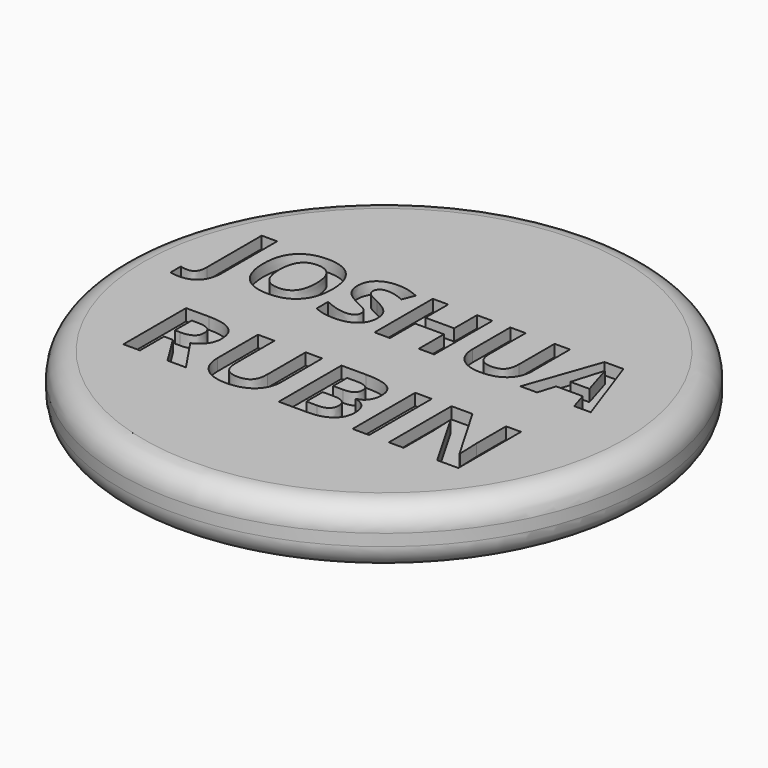
from build123d import *

# Parameters (mm, degrees)
F0_R           = 57.15
F1_DEPTH       = 12.7
F2_R           = 5.08
F3_TEXT_SIZE   = 22.0706776834
F3_TEXT_SIZE_2 = 23.7602923264
F4_DEPTH       = 2.54


# Not quite as in the source:
# - Text() gives the source's letters only with a copy of the font that has no kerning and outlines rounded to 1/6400 em; it was checked with that copy


with BuildPart() as f1:
    # F0 (on Top) → F1 (new body)
    with BuildSketch(Plane.XY):
        Circle(F0_R)
    extrude(amount=F1_DEPTH)

    # F2
    f2_edges = [f1.edges().sort_by_distance(p)[0] for p in [
        (-57.15, 0, 12.7),
        (-57.15, 0, 0),
    ]]
    fillet(f2_edges, radius=F2_R)

    # F3 (on face) → F4 (cut)
    with BuildSketch(Plane.XY.offset(12.7)):
        with Locations((-44.45, 4.2110964911)):
            Text('JOSHUA', F3_TEXT_SIZE, font='Open Sans', font_style=FontStyle.BOLD, text_align=(TextAlign.LEFT, TextAlign.BOTTOM))
        with Locations((-38.0133874714, -25.7134122098)):
            Text('RUBIN', F3_TEXT_SIZE_2, font='Open Sans', font_style=FontStyle.BOLD, text_align=(TextAlign.LEFT, TextAlign.BOTTOM))
    extrude(amount=-F4_DEPTH, mode=Mode.SUBTRACT)


solid = f1.part
